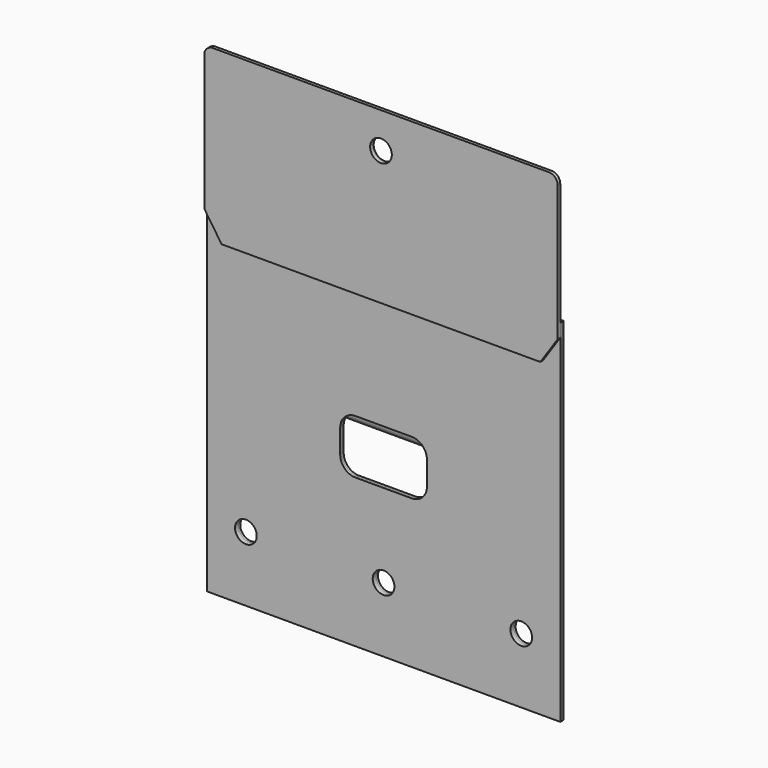
from build123d import *

# Parameters (mm, degrees)
F1_DEPTH = 5
F2_R     = 4.5
F3_W     = 163
F3_H     = 162
F3_R     = 5
F4_DEPTH = 2
F5_DEPTH = 1
F6_R     = 5
F7_DEPTH = 1.5
F8_DEPTH = 0.55
F9_DEPTH = 1


# Not quite as in the source:
# - a feature names something its author has since deleted; it is built from what else it names


with BuildPart() as f1:
    # F0 (on Front) → F1 (new body, symmetric)
    with BuildSketch(Plane.XZ):
        with BuildLine():
            ThreePointArc((73.5, 28), (71.1568542495, 33.6568542495), (65.5, 36))
            Line((65.5, 36), (-65.5, 36))
            ThreePointArc((-65.5, 36), (-71.1568542495, 33.6568542495), (-73.5, 28))
            Line((-73.5, 28), (-73.5, -28))
            ThreePointArc((-73.5, -28), (-71.1568542495, -33.6568542495), (-65.5, -36))
            Line((-65.5, -36), (65.5, -36))
            ThreePointArc((65.5, -36), (71.1568542495, -33.6568542495), (73.5, -28))
            Line((73.5, -28), (73.5, 28))
        make_face()
    extrude(amount=F1_DEPTH, both=True)

    # F2
    f2_edges = [f1.edges().sort_by_distance(p)[0] for p in [
        (71.156854, -5, 33.656854),
        (0, -5, 36),
        (-71.156854, -5, 33.656854),
        (-73.5, -5, 0),
        (-71.156854, -5, -33.656854),
        (0, -5, -36),
        (71.156854, -5, -33.656854),
        (73.5, -5, 0),
        (71.156854, 5, 33.656854),
        (0, 5, 36),
        (-71.156854, 5, 33.656854),
        (-73.5, 5, 0),
        (-71.156854, 5, -33.656854),
        (0, 5, -36),
        (71.156854, 5, -33.656854),
        (73.5, 5, 0),
    ]]
    fillet(f2_edges, radius=F2_R)


with BuildPart() as f4:
    # F3 (on face) → F4 (new body)
    with BuildSketch(Plane.XZ.offset(5)):
        with Locations((0, -43)):
            Rectangle(F3_W, F3_H)
        with BuildLine():
            Line((-73.5, -50), (-24.9058808998, -50))
            ThreePointArc((-24.9058808998, -50), (-20.9372539332, -57.5), (-13, -60.5))
            Line((-13, -60.5), (13, -60.5))
            ThreePointArc((13, -60.5), (20.9372539332, -57.5), (24.9058808998, -50))
            Line((24.9058808998, -50), (73.5, -50))
            Line((73.5, -50), (73.5, -118))
            Line((73.5, -118), (-73.5, -118))
            Line((-73.5, -118), (-73.5, -50))
        make_face(mode=Mode.SUBTRACT)
        with BuildLine():
            ThreePointArc((-20, -37.5), (-17.9497474683, -32.5502525317), (-13, -30.5))
            Line((-13, -30.5), (13, -30.5))
            ThreePointArc((13, -30.5), (17.9497474683, -32.5502525317), (20, -37.5))
            Line((20, -37.5), (20, -48.5))
            ThreePointArc((20, -48.5), (17.9497474683, -53.4497474683), (13, -55.5))
            Line((13, -55.5), (-13, -55.5))
            ThreePointArc((-13, -55.5), (-17.9497474683, -53.4497474683), (-20, -48.5))
            Line((-20, -48.5), (-20, -37.5))
        make_face(mode=Mode.SUBTRACT)
        with BuildLine():
            Line((73.5, 32), (73.5, -36))
            Line((73.5, -36), (24.9058808998, -36))
            ThreePointArc((24.9058808998, -36), (20.9372539332, -28.5), (13, -25.5))
            Line((13, -25.5), (-13, -25.5))
            ThreePointArc((-13, -25.5), (-20.9372539332, -28.5), (-24.9058808998, -36))
            Line((-24.9058808998, -36), (-73.5, -36))
            Line((-73.5, -36), (-73.5, 32))
            Line((-73.5, 32), (73.5, 32))
        make_face(mode=Mode.SUBTRACT)
        with BuildLine():
            ThreePointArc((13, -25.5), (19, -27.1076951546), (23.3923048454, -31.5))
            Line((23.3923048454, -31.5), (65.5, -31.5))
            ThreePointArc((65.5, -31.5), (67.9748737342, -30.4748737342), (69, -28))
            Line((69, -28), (69, 28))
            ThreePointArc((69, 28), (67.9748737342, 30.4748737342), (65.5, 31.5))
            Line((65.5, 31.5), (-65.5, 31.5))
            ThreePointArc((-65.5, 31.5), (-67.9748737342, 30.4748737342), (-69, 28))
            Line((-69, 28), (-69, -28))
            ThreePointArc((-69, -28), (-67.9748737342, -30.4748737342), (-65.5, -31.5))
            Line((-65.5, -31.5), (-23.3923048454, -31.5))
            ThreePointArc((-23.3923048454, -31.5), (-19, -27.1076951546), (-13, -25.5))
            Line((-13, -25.5), (13, -25.5))
        make_face()
        with BuildLine():
            ThreePointArc((-13, -60.5), (-20.9372539332, -57.5), (-24.9058808998, -50))
            Line((-24.9058808998, -50), (-73.5, -50))
            Line((-73.5, -50), (-73.5, -118))
            Line((-73.5, -118), (73.5, -118))
            Line((73.5, -118), (73.5, -50))
            Line((73.5, -50), (24.9058808998, -50))
            ThreePointArc((24.9058808998, -50), (20.9372539332, -57.5), (13, -60.5))
            Line((13, -60.5), (-13, -60.5))
        make_face()
        with Locations((-63.5, -94)):
            Circle(F3_R, mode=Mode.SUBTRACT)
        with Locations((0, -94)):
            Circle(F3_R, mode=Mode.SUBTRACT)
        with Locations((63.5, -94)):
            Circle(F3_R, mode=Mode.SUBTRACT)
        with BuildLine():
            Line((24.9058808998, -36), (73.5, -36))
            Line((73.5, -36), (73.5, 32))
            Line((73.5, 32), (-73.5, 32))
            Line((-73.5, 32), (-73.5, -36))
            Line((-73.5, -36), (-24.9058808998, -36))
            ThreePointArc((-24.9058808998, -36), (-24.3738635424, -33.6743983325), (-23.3923048454, -31.5))
            Line((-23.3923048454, -31.5), (-65.5, -31.5))
            ThreePointArc((-65.5, -31.5), (-67.9748737342, -30.4748737342), (-69, -28))
            Line((-69, -28), (-69, 28))
            ThreePointArc((-69, 28), (-67.9748737342, 30.4748737342), (-65.5, 31.5))
            Line((-65.5, 31.5), (65.5, 31.5))
            ThreePointArc((65.5, 31.5), (67.9748737342, 30.4748737342), (69, 28))
            Line((69, 28), (69, -28))
            ThreePointArc((69, -28), (67.9748737342, -30.4748737342), (65.5, -31.5))
            Line((65.5, -31.5), (23.3923048454, -31.5))
            ThreePointArc((23.3923048454, -31.5), (24.3738635424, -33.6743983325), (24.9058808998, -36))
        make_face()
    extrude(amount=F4_DEPTH)


with BuildPart() as f5:
    # F3 (on face) → F5 (new body)
    with BuildSketch(Plane.XZ.offset(5)):
        with BuildLine():
            Line((24.9058808998, -36), (73.5, -36))
            Line((73.5, -36), (73.5, 32))
            Line((73.5, 32), (-73.5, 32))
            Line((-73.5, 32), (-73.5, -36))
            Line((-73.5, -36), (-24.9058808998, -36))
            ThreePointArc((-24.9058808998, -36), (-24.3738635424, -33.6743983325), (-23.3923048454, -31.5))
            Line((-23.3923048454, -31.5), (-65.5, -31.5))
            ThreePointArc((-65.5, -31.5), (-67.9748737342, -30.4748737342), (-69, -28))
            Line((-69, -28), (-69, 28))
            ThreePointArc((-69, 28), (-67.9748737342, 30.4748737342), (-65.5, 31.5))
            Line((-65.5, 31.5), (65.5, 31.5))
            ThreePointArc((65.5, 31.5), (67.9748737342, 30.4748737342), (69, 28))
            Line((69, 28), (69, -28))
            ThreePointArc((69, -28), (67.9748737342, -30.4748737342), (65.5, -31.5))
            Line((65.5, -31.5), (23.3923048454, -31.5))
            ThreePointArc((23.3923048454, -31.5), (24.3738635424, -33.6743983325), (24.9058808998, -36))
        make_face()
        with BuildLine():
            ThreePointArc((13, -25.5), (19, -27.1076951546), (23.3923048454, -31.5))
            Line((23.3923048454, -31.5), (65.5, -31.5))
            ThreePointArc((65.5, -31.5), (67.9748737342, -30.4748737342), (69, -28))
            Line((69, -28), (69, 28))
            ThreePointArc((69, 28), (67.9748737342, 30.4748737342), (65.5, 31.5))
            Line((65.5, 31.5), (-65.5, 31.5))
            ThreePointArc((-65.5, 31.5), (-67.9748737342, 30.4748737342), (-69, 28))
            Line((-69, 28), (-69, -28))
            ThreePointArc((-69, -28), (-67.9748737342, -30.4748737342), (-65.5, -31.5))
            Line((-65.5, -31.5), (-23.3923048454, -31.5))
            ThreePointArc((-23.3923048454, -31.5), (-19, -27.1076951546), (-13, -25.5))
            Line((-13, -25.5), (13, -25.5))
        make_face()
    extrude(amount=-F5_DEPTH)


with BuildPart() as f5b:
    # F3 (on face) → F5, piece 2 (new body)
    with BuildSketch(Plane.XZ.offset(5)):
        with BuildLine():
            ThreePointArc((-13, -60.5), (-20.9372539332, -57.5), (-24.9058808998, -50))
            Line((-24.9058808998, -50), (-73.5, -50))
            Line((-73.5, -50), (-73.5, -118))
            Line((-73.5, -118), (73.5, -118))
            Line((73.5, -118), (73.5, -50))
            Line((73.5, -50), (24.9058808998, -50))
            ThreePointArc((24.9058808998, -50), (20.9372539332, -57.5), (13, -60.5))
            Line((13, -60.5), (-13, -60.5))
        make_face()
        with Locations((-63.5, -94)):
            Circle(F3_R, mode=Mode.SUBTRACT)
        with Locations((0, -94)):
            Circle(F3_R, mode=Mode.SUBTRACT)
        with Locations((63.5, -94)):
            Circle(F3_R, mode=Mode.SUBTRACT)
    extrude(amount=-F5_DEPTH)


with BuildPart() as f7:
    # F6 (on face) → F7 (new body)
    with BuildSketch(Plane.XZ.offset(7)):
        with BuildLine():
            ThreePointArc((-77.5, 98.496), (-80.3284271247, 97.3244271247), (-81.5, 94.496))
            Line((-81.5, 94.496), (-81.5, 38))
            Line((-81.5, 38), (81.5, 38))
            Line((81.5, 38), (81.5, 94.496))
            ThreePointArc((81.5, 94.496), (80.3284271247, 97.3244271247), (77.5, 98.496))
            Line((77.5, 98.496), (0, 98.496))
            Line((0, 98.496), (-77.5, 98.496))
        make_face()
        with BuildLine():
            Line((73.5, 54), (-73.5, 54))
            Line((-73.5, 54), (-73.5, 92.996))
            ThreePointArc((-73.5, 92.996), (-73.0606601718, 94.0566601718), (-72, 94.496))
            Line((-72, 94.496), (72, 94.496))
            ThreePointArc((72, 94.496), (73.0606601718, 94.0566601718), (73.5, 92.996))
            Line((73.5, 92.996), (73.5, 54))
        make_face(mode=Mode.SUBTRACT)
        Polygon((81.5, 38), (-81.5, 38), (-81.5, 32), (-73.5, 20.16), (0, 20.16), (73.5, 20.16), (81.5, 32), align=None)
        with BuildLine():
            Line((-73.5, 92.996), (-73.5, 54))
            Line((-73.5, 54), (73.5, 54))
            Line((73.5, 54), (73.5, 92.996))
            ThreePointArc((73.5, 92.996), (73.0606601718, 94.0566601718), (72, 94.496))
            Line((72, 94.496), (-72, 94.496))
            ThreePointArc((-72, 94.496), (-73.0606601718, 94.0566601718), (-73.5, 92.996))
        make_face()
        with Locations((-63.5, 82)):
            Circle(F6_R, mode=Mode.SUBTRACT)
        with Locations((0, 82)):
            Circle(F6_R, mode=Mode.SUBTRACT)
        with Locations((63.5, 82)):
            Circle(F6_R, mode=Mode.SUBTRACT)
        with Locations((63.5, 82)):
            Circle(F6_R)
        with Locations((-63.5, 82)):
            Circle(F6_R)
    extrude(amount=F7_DEPTH)


with BuildPart() as f8:
    # F6 (on face) → F8 (new body)
    with BuildSketch(Plane.XZ.offset(7)):
        with BuildLine():
            Line((-73.5, 92.996), (-73.5, 54))
            Line((-73.5, 54), (73.5, 54))
            Line((73.5, 54), (73.5, 92.996))
            ThreePointArc((73.5, 92.996), (73.0606601718, 94.0566601718), (72, 94.496))
            Line((72, 94.496), (-72, 94.496))
            ThreePointArc((-72, 94.496), (-73.0606601718, 94.0566601718), (-73.5, 92.996))
        make_face()
        with Locations((-63.5, 82)):
            Circle(F6_R, mode=Mode.SUBTRACT)
        with Locations((0, 82)):
            Circle(F6_R, mode=Mode.SUBTRACT)
        with Locations((63.5, 82)):
            Circle(F6_R, mode=Mode.SUBTRACT)
    extrude(amount=-F8_DEPTH)


with BuildPart() as f9:
    # F3 (on face) → F9 (new body)
    with BuildSketch(Plane.XZ.offset(5)):
        with Locations((0, -43)):
            Rectangle(F3_W, F3_H)
        with BuildLine():
            Line((-73.5, -50), (-24.9058808998, -50))
            ThreePointArc((-24.9058808998, -50), (-20.9372539332, -57.5), (-13, -60.5))
            Line((-13, -60.5), (13, -60.5))
            ThreePointArc((13, -60.5), (20.9372539332, -57.5), (24.9058808998, -50))
            Line((24.9058808998, -50), (73.5, -50))
            Line((73.5, -50), (73.5, -118))
            Line((73.5, -118), (-73.5, -118))
            Line((-73.5, -118), (-73.5, -50))
        make_face(mode=Mode.SUBTRACT)
        with BuildLine():
            ThreePointArc((-20, -37.5), (-17.9497474683, -32.5502525317), (-13, -30.5))
            Line((-13, -30.5), (13, -30.5))
            ThreePointArc((13, -30.5), (17.9497474683, -32.5502525317), (20, -37.5))
            Line((20, -37.5), (20, -48.5))
            ThreePointArc((20, -48.5), (17.9497474683, -53.4497474683), (13, -55.5))
            Line((13, -55.5), (-13, -55.5))
            ThreePointArc((-13, -55.5), (-17.9497474683, -53.4497474683), (-20, -48.5))
            Line((-20, -48.5), (-20, -37.5))
        make_face(mode=Mode.SUBTRACT)
        with BuildLine():
            Line((73.5, 32), (73.5, -36))
            Line((73.5, -36), (24.9058808998, -36))
            ThreePointArc((24.9058808998, -36), (20.9372539332, -28.5), (13, -25.5))
            Line((13, -25.5), (-13, -25.5))
            ThreePointArc((-13, -25.5), (-20.9372539332, -28.5), (-24.9058808998, -36))
            Line((-24.9058808998, -36), (-73.5, -36))
            Line((-73.5, -36), (-73.5, 32))
            Line((-73.5, 32), (73.5, 32))
        make_face(mode=Mode.SUBTRACT)
        with BuildLine():
            Line((24.9058808998, -36), (73.5, -36))
            Line((73.5, -36), (73.5, 32))
            Line((73.5, 32), (-73.5, 32))
            Line((-73.5, 32), (-73.5, -36))
            Line((-73.5, -36), (-24.9058808998, -36))
            ThreePointArc((-24.9058808998, -36), (-24.3738635424, -33.6743983325), (-23.3923048454, -31.5))
            Line((-23.3923048454, -31.5), (-65.5, -31.5))
            ThreePointArc((-65.5, -31.5), (-67.9748737342, -30.4748737342), (-69, -28))
            Line((-69, -28), (-69, 28))
            ThreePointArc((-69, 28), (-67.9748737342, 30.4748737342), (-65.5, 31.5))
            Line((-65.5, 31.5), (65.5, 31.5))
            ThreePointArc((65.5, 31.5), (67.9748737342, 30.4748737342), (69, 28))
            Line((69, 28), (69, -28))
            ThreePointArc((69, -28), (67.9748737342, -30.4748737342), (65.5, -31.5))
            Line((65.5, -31.5), (23.3923048454, -31.5))
            ThreePointArc((23.3923048454, -31.5), (24.3738635424, -33.6743983325), (24.9058808998, -36))
        make_face()
        with BuildLine():
            ThreePointArc((13, -25.5), (19, -27.1076951546), (23.3923048454, -31.5))
            Line((23.3923048454, -31.5), (65.5, -31.5))
            ThreePointArc((65.5, -31.5), (67.9748737342, -30.4748737342), (69, -28))
            Line((69, -28), (69, 28))
            ThreePointArc((69, 28), (67.9748737342, 30.4748737342), (65.5, 31.5))
            Line((65.5, 31.5), (-65.5, 31.5))
            ThreePointArc((-65.5, 31.5), (-67.9748737342, 30.4748737342), (-69, 28))
            Line((-69, 28), (-69, -28))
            ThreePointArc((-69, -28), (-67.9748737342, -30.4748737342), (-65.5, -31.5))
            Line((-65.5, -31.5), (-23.3923048454, -31.5))
            ThreePointArc((-23.3923048454, -31.5), (-19, -27.1076951546), (-13, -25.5))
            Line((-13, -25.5), (13, -25.5))
        make_face()
    extrude(amount=F9_DEPTH)


solid = Compound([f1.part, f4.part, f5.part, f5b.part, f7.part, f8.part, f9.part])
